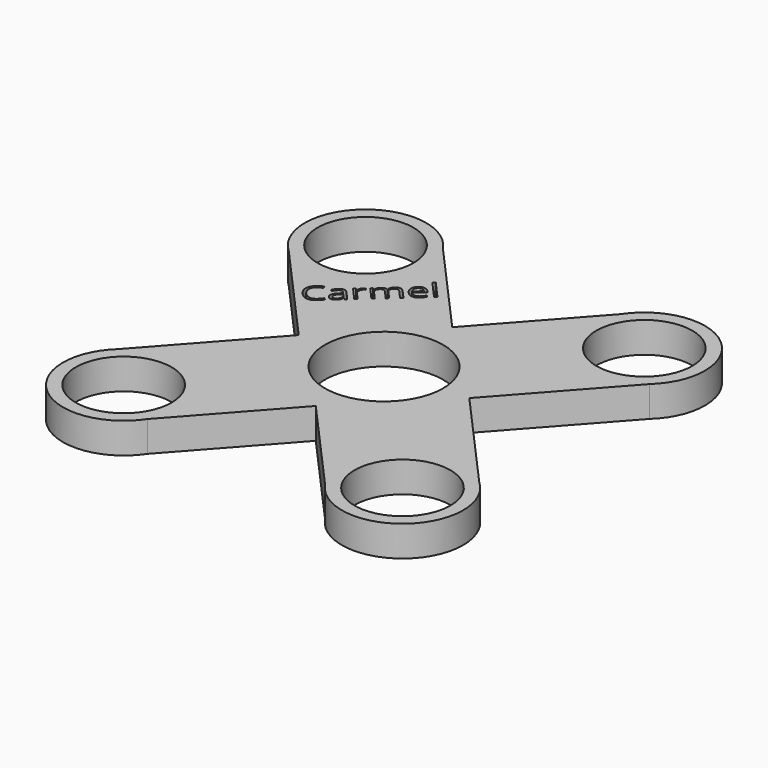
from build123d import *

# Parameters (mm, degrees)
F0_R         = 15.3905754666
F0_R_2       = 12.5
F1_DEPTH     = 8
F2_TEXT_SIZE = 8.5685505635
F3_DEPTH     = 11.5


# Not quite as in the source:
# - Text() gives the source's letters only with a copy of the font that has no kerning and outlines rounded to 1/6400 em; it was checked with that copy


with BuildPart() as f1:
    # F0 (on Top) → F1 (new body)
    with BuildSketch(Plane.XY):
        with BuildLine():
            ThreePointArc((0, -22.2422045564), (15.7276136703, -15.7276136703), (22.2422045564, 0))
            ThreePointArc((22.2422045564, 0), (15.7276136703, 15.7276136703), (0, 22.2422045564))
            ThreePointArc((0, 22.2422045564), (-15.7276136703, 15.7276136703), (-22.2422045564, 0))
            ThreePointArc((-22.2422045564, 0), (-15.7276136703, -15.7276136703), (0, -22.2422045564))
        make_face()
        Circle(F0_R, mode=Mode.SUBTRACT)
        with BuildLine():
            Line((47.051167809, -27.7575870879), (22.2422045564, 0))
            ThreePointArc((22.2422045564, 0), (15.7276136703, -15.7276136703), (0, -22.2422045564))
            Line((0, -22.2422045564), (23.1625940977, -48.1577463024))
            ThreePointArc((23.1625940977, -48.1577463024), (46.629287134, -51.4503971432), (47.051167809, -27.7575870879))
        make_face()
        with Locations((36.3533315535, -39.4172595702)):
            Circle(F0_R_2, mode=Mode.SUBTRACT)
        with BuildLine():
            ThreePointArc((0, 22.2422045564), (15.7276136703, 15.7276136703), (22.2422045564, 0))
            Line((22.2422045564, 0), (47.051167809, 27.7575870879))
            ThreePointArc((47.051167809, 27.7575870879), (46.629287134, 51.4503971432), (23.1625940977, 48.1577463024))
            Line((23.1625940977, 48.1577463024), (0, 22.2422045564))
        make_face()
        with Locations((36.3533315535, 39.4172595702)):
            Circle(F0_R_2, mode=Mode.SUBTRACT)
        with BuildLine():
            ThreePointArc((-22.2422045564, 0), (-15.7276136703, 15.7276136703), (0, 22.2422045564))
            Line((0, 22.2422045564), (-23.1625940977, 48.1577463024))
            ThreePointArc((-23.1625940977, 48.1577463024), (-46.629287134, 51.4503971432), (-47.051167809, 27.7575870879))
            Line((-47.051167809, 27.7575870879), (-22.2422045564, 0))
        make_face()
        with Locations((-36.3533315535, 39.4172595702)):
            Circle(F0_R_2, mode=Mode.SUBTRACT)
        with BuildLine():
            Line((-23.1625940977, -48.1577463024), (0, -22.2422045564))
            ThreePointArc((0, -22.2422045564), (-15.7276136703, -15.7276136703), (-22.2422045564, 0))
            Line((-22.2422045564, 0), (-47.051167809, -27.7575870879))
            ThreePointArc((-47.051167809, -27.7575870879), (-46.629287134, -51.4503971432), (-23.1625940977, -48.1577463024))
        make_face()
        with Locations((-36.3533315535, -39.4172595702)):
            Circle(F0_R_2, mode=Mode.SUBTRACT)
    extrude(amount=F1_DEPTH)

    # F2 (on Top) → F3 (cut)
    with BuildSketch(Plane.XY):
        with Locations(Location((-31.4532870913, 12.1844135386), (0, 0, 41.7894631993))):
            Text('Carmel', F2_TEXT_SIZE, font='Open Sans', text_align=(TextAlign.LEFT, TextAlign.BOTTOM))
    extrude(amount=F3_DEPTH, mode=Mode.SUBTRACT)


solid = f1.part
